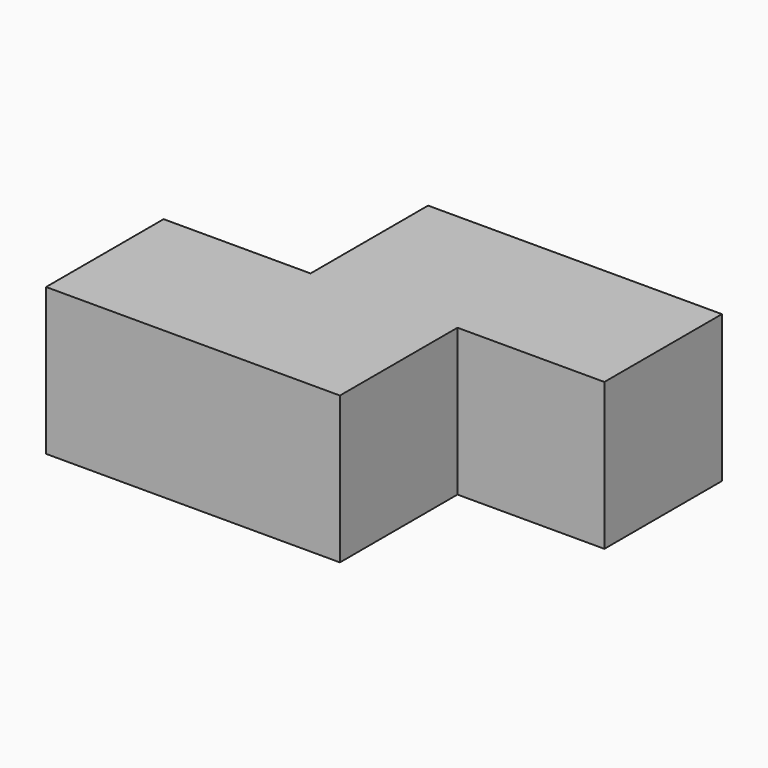
from build123d import *

# Parameters (mm, degrees)
F1_W     = 76.2
F1_H     = 50.8
F2_DEPTH = 25.4
F3_W     = 25.4
F3_H     = 25.4
F4_DEPTH = 25.4
F5_W     = 25.4
F5_H     = 25.4
F6_DEPTH = 25.4


# Not quite as in the source:
# - a variable given as a bare number and used for a length is read in inches; the dataset says mm whatever the document's units were


with BuildPart() as f2:
    # F1 (on Top) → F2 (new body)
    with BuildSketch(Plane.XY):
        Rectangle(F1_W, F1_H)
    extrude(amount=F2_DEPTH)

    # F3 (on face) → F4 (cut)
    with BuildSketch(Plane.XY.offset(25.4)):
        with Locations((-25.4, 12.7)):
            Rectangle(F3_W, F3_H)
    extrude(amount=-F4_DEPTH, mode=Mode.SUBTRACT)

    # F5 (on face) → F6 (cut)
    with BuildSketch(Plane.XY.offset(25.4)):
        with Locations((25.4, -12.7)):
            Rectangle(F5_W, F5_H)
    extrude(amount=-F6_DEPTH, mode=Mode.SUBTRACT)


solid = f2.part
